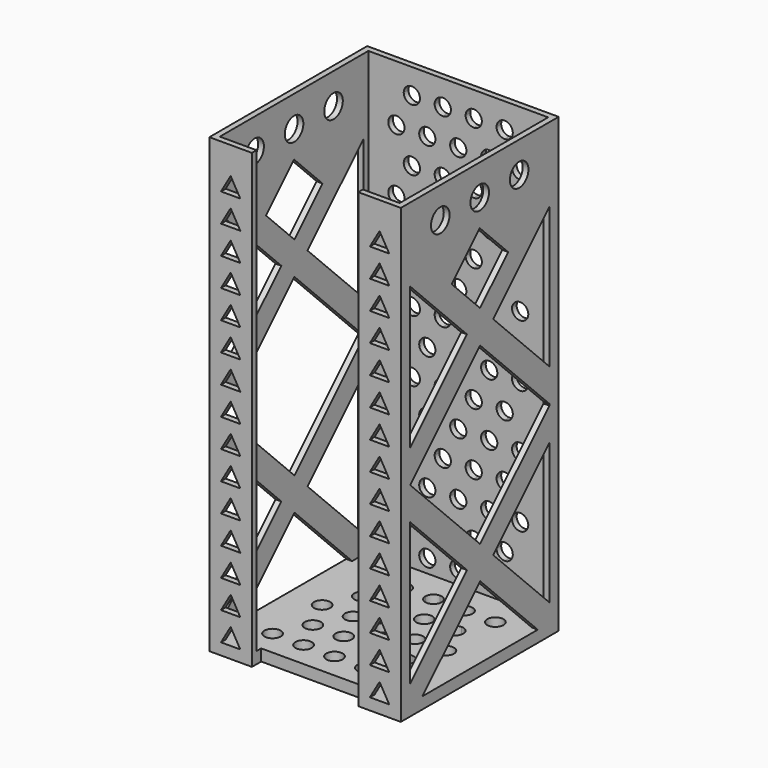
from build123d import *

# Parameters (mm, degrees)
F0_W      = 49.5
F0_H      = 51
F1_DEPTH  = 3
F2_W      = 49.5
F2_H      = 51
F2_W_2    = 46.5
F2_H_2    = 48
F3_DEPTH  = 114
F4_W      = 27.5
F4_H      = 117
F5_DEPTH  = 3
F6_R      = 2.1
F7_DEPTH  = 3
F9_DEPTH  = 106.1
F11_DEPTH = 49.501
F12_R     = 2.1
F13_DEPTH = 4
F15_DEPTH = 25


# Not quite as in the source:
# - ends of sketch curves that miss each other by under 0.0002 mm in the source are joined


with BuildPart() as f1:
    # F0 (on Top) → F1 (new body)
    with BuildSketch(Plane.XY):
        Rectangle(F0_W, F0_H)
    extrude(amount=F1_DEPTH)

    # F2 (on face) → F3 (join)
    with BuildSketch(Plane.XY.offset(3)):
        Rectangle(F2_W, F2_H)
        Rectangle(F2_W_2, F2_H_2, mode=Mode.SUBTRACT)
    extrude(amount=F3_DEPTH)

    # F4 (on face) → F5 (cut)
    with BuildSketch(Plane.XZ.offset(25.5)):
        with Locations((0, 58.5)):
            Rectangle(F4_W, F4_H)
    extrude(amount=-F5_DEPTH, mode=Mode.SUBTRACT)

    # F6 (on face) → F7 (cut)
    with BuildSketch(Plane(origin=(0, 25.5, 0), x_dir=(-1, 0, 0), z_dir=(0, 1, 0))):
        with Locations((-16, 6.5)):
            Circle(F6_R)
        with BuildLine():
            ThreePointArc((18.1, 6.5), (16, 8.6), (13.9, 6.5))
            ThreePointArc((13.9, 6.5), (16, 4.4), (18.1, 6.5))
        make_face()
        with BuildLine():
            ThreePointArc((-9.9, 14.5), (-13.4849242405, 15.9849242405), (-12, 12.4))
            ThreePointArc((-12, 12.4), (-10.5150757595, 13.0150757595), (-9.9, 14.5))
        make_face()
        with BuildLine():
            ThreePointArc((-1.9, 14.5), (-5.4849242405, 15.9849242405), (-4, 12.4))
            ThreePointArc((-4, 12.4), (-2.5150757595, 13.0150757595), (-1.9, 14.5))
        make_face()
        with BuildLine():
            ThreePointArc((6.1, 14.5), (2.5150757595, 15.9849242405), (4, 12.4))
            ThreePointArc((4, 12.4), (5.4849242405, 13.0150757595), (6.1, 14.5))
        make_face()
        with BuildLine():
            ThreePointArc((14.1, 14.5), (10.5150757595, 15.9849242405), (12, 12.4))
            ThreePointArc((12, 12.4), (13.4849242405, 13.0150757595), (14.1, 14.5))
        make_face()
        with BuildLine():
            ThreePointArc((12, 28.4), (13.4849242405, 29.0150757595), (14.1, 30.5))
            ThreePointArc((14.1, 30.5), (10.5150757595, 31.9849242405), (12, 28.4))
        make_face()
        with BuildLine():
            ThreePointArc((-1.9, 30.5), (-5.4849242405, 31.9849242405), (-4, 28.4))
            ThreePointArc((-4, 28.4), (-2.5150757595, 29.0150757595), (-1.9, 30.5))
        make_face()
        with BuildLine():
            ThreePointArc((-9.9, 30.5), (-13.4849242405, 31.9849242405), (-12, 28.4))
            ThreePointArc((-12, 28.4), (-10.5150757595, 29.0150757595), (-9.9, 30.5))
        make_face()
        with Locations((-16, 22.5)):
            Circle(F6_R)
        with BuildLine():
            ThreePointArc((6.1, 30.5), (2.5150757595, 31.9849242405), (4, 28.4))
            ThreePointArc((4, 28.4), (5.4849242405, 29.0150757595), (6.1, 30.5))
        make_face()
        with BuildLine():
            ThreePointArc((18.1, 22.5), (16, 24.6), (13.9, 22.5))
            ThreePointArc((13.9, 22.5), (16, 20.4), (18.1, 22.5))
        make_face()
        with BuildLine():
            ThreePointArc((12, 44.4), (13.4849242405, 45.0150757595), (14.1, 46.5))
            ThreePointArc((14.1, 46.5), (10.5150757595, 47.9849242405), (12, 44.4))
        make_face()
        with BuildLine():
            ThreePointArc((-1.9, 46.5), (-5.4849242405, 47.9849242405), (-4, 44.4))
            ThreePointArc((-4, 44.4), (-2.5150757595, 45.0150757595), (-1.9, 46.5))
        make_face()
        with BuildLine():
            ThreePointArc((-9.9, 46.5), (-13.4849242405, 47.9849242405), (-12, 44.4))
            ThreePointArc((-12, 44.4), (-10.5150757595, 45.0150757595), (-9.9, 46.5))
        make_face()
        with Locations((-16, 38.5)):
            Circle(F6_R)
        with BuildLine():
            ThreePointArc((6.1, 46.5), (2.5150757595, 47.9849242405), (4, 44.4))
            ThreePointArc((4, 44.4), (5.4849242405, 45.0150757595), (6.1, 46.5))
        make_face()
        with BuildLine():
            ThreePointArc((18.1, 38.5), (16, 40.6), (13.9, 38.5))
            ThreePointArc((13.9, 38.5), (16, 36.4), (18.1, 38.5))
        make_face()
        with BuildLine():
            ThreePointArc((12, 60.4), (13.4849242405, 61.0150757595), (14.1, 62.5))
            ThreePointArc((14.1, 62.5), (10.5150757595, 63.9849242405), (12, 60.4))
        make_face()
        with BuildLine():
            ThreePointArc((-1.9, 62.5), (-5.4849242405, 63.9849242405), (-4, 60.4))
            ThreePointArc((-4, 60.4), (-2.5150757595, 61.0150757595), (-1.9, 62.5))
        make_face()
        with BuildLine():
            ThreePointArc((-9.9, 62.5), (-13.4849242405, 63.9849242405), (-12, 60.4))
            ThreePointArc((-12, 60.4), (-10.5150757595, 61.0150757595), (-9.9, 62.5))
        make_face()
        with Locations((-16, 54.5)):
            Circle(F6_R)
        with BuildLine():
            ThreePointArc((6.1, 62.5), (2.5150757595, 63.9849242405), (4, 60.4))
            ThreePointArc((4, 60.4), (5.4849242405, 61.0150757595), (6.1, 62.5))
        make_face()
        with BuildLine():
            ThreePointArc((18.1, 54.5), (16, 56.6), (13.9, 54.5))
            ThreePointArc((13.9, 54.5), (16, 52.4), (18.1, 54.5))
        make_face()
        with BuildLine():
            ThreePointArc((12, 76.4), (13.4849242405, 77.0150757595), (14.1, 78.5))
            ThreePointArc((14.1, 78.5), (10.5150757595, 79.9849242405), (12, 76.4))
        make_face()
        with BuildLine():
            ThreePointArc((-1.9, 78.5), (-5.4849242405, 79.9849242405), (-4, 76.4))
            ThreePointArc((-4, 76.4), (-2.5150757595, 77.0150757595), (-1.9, 78.5))
        make_face()
        with BuildLine():
            ThreePointArc((-9.9, 78.5), (-13.4849242405, 79.9849242405), (-12, 76.4))
            ThreePointArc((-12, 76.4), (-10.5150757595, 77.0150757595), (-9.9, 78.5))
        make_face()
        with Locations((-16, 70.5)):
            Circle(F6_R)
        with BuildLine():
            ThreePointArc((6.1, 78.5), (2.5150757595, 79.9849242405), (4, 76.4))
            ThreePointArc((4, 76.4), (5.4849242405, 77.0150757595), (6.1, 78.5))
        make_face()
        with BuildLine():
            ThreePointArc((18.1, 70.5), (16, 72.6), (13.9, 70.5))
            ThreePointArc((13.9, 70.5), (16, 68.4), (18.1, 70.5))
        make_face()
        with BuildLine():
            ThreePointArc((12, 92.4), (13.4849242405, 93.0150757595), (14.1, 94.5))
            ThreePointArc((14.1, 94.5), (10.5150757595, 95.9849242405), (12, 92.4))
        make_face()
        with BuildLine():
            ThreePointArc((-1.9, 94.5), (-5.4849242405, 95.9849242405), (-4, 92.4))
            ThreePointArc((-4, 92.4), (-2.5150757595, 93.0150757595), (-1.9, 94.5))
        make_face()
        with BuildLine():
            ThreePointArc((-9.9, 94.5), (-13.4849242405, 95.9849242405), (-12, 92.4))
            ThreePointArc((-12, 92.4), (-10.5150757595, 93.0150757595), (-9.9, 94.5))
        make_face()
        with Locations((-16, 86.5)):
            Circle(F6_R)
        with BuildLine():
            ThreePointArc((6.1, 94.5), (2.5150757595, 95.9849242405), (4, 92.4))
            ThreePointArc((4, 92.4), (5.4849242405, 93.0150757595), (6.1, 94.5))
        make_face()
        with BuildLine():
            ThreePointArc((18.1, 86.5), (16, 88.6), (13.9, 86.5))
            ThreePointArc((13.9, 86.5), (16, 84.4), (18.1, 86.5))
        make_face()
        with BuildLine():
            ThreePointArc((14.1, 110.5), (10.5150757595, 111.9849242405), (12, 108.4))
            ThreePointArc((12, 108.4), (13.4849242405, 109.0150757595), (14.1, 110.5))
        make_face()
        with BuildLine():
            ThreePointArc((-9.9, 110.5), (-13.4849242405, 111.9849242405), (-12, 108.4))
            ThreePointArc((-12, 108.4), (-10.5150757595, 109.0150757595), (-9.9, 110.5))
        make_face()
        with Locations((-16, 102.5)):
            Circle(F6_R)
        with BuildLine():
            ThreePointArc((18.1, 102.5), (16, 104.6), (13.9, 102.5))
            ThreePointArc((13.9, 102.5), (16, 100.4), (18.1, 102.5))
        make_face()
        with BuildLine():
            Line((-8, 6.5), (-5.9, 6.5))
            ThreePointArc((-5.9, 6.5), (-8, 8.6), (-10.1, 6.5))
            Line((-10.1, 6.5), (-8, 6.5))
        make_face()
        with BuildLine():
            ThreePointArc((-10.1, 6.5), (-8, 4.4), (-5.9, 6.5))
            Line((-5.9, 6.5), (-8, 6.5))
            Line((-8, 6.5), (-10.1, 6.5))
        make_face()
        with BuildLine():
            ThreePointArc((10.1, 6.5), (8, 8.6), (5.9, 6.5))
            Line((5.9, 6.5), (8, 6.5))
            Line((8, 6.5), (10.1, 6.5))
        make_face()
        with BuildLine():
            Line((8, 6.5), (5.9, 6.5))
            ThreePointArc((5.9, 6.5), (8, 4.4), (10.1, 6.5))
            Line((10.1, 6.5), (8, 6.5))
        make_face()
        with BuildLine():
            Line((-8, 22.5), (-5.9, 22.5))
            ThreePointArc((-5.9, 22.5), (-8, 24.6), (-10.1, 22.5))
            Line((-10.1, 22.5), (-8, 22.5))
        make_face()
        with BuildLine():
            ThreePointArc((-10.1, 22.5), (-8, 20.4), (-5.9, 22.5))
            Line((-5.9, 22.5), (-8, 22.5))
            Line((-8, 22.5), (-10.1, 22.5))
        make_face()
        with BuildLine():
            Line((8, 22.5), (10.1, 22.5))
            ThreePointArc((10.1, 22.5), (8, 24.6), (5.9, 22.5))
            Line((5.9, 22.5), (8, 22.5))
        make_face()
        with BuildLine():
            ThreePointArc((5.9, 22.5), (8, 20.4), (10.1, 22.5))
            Line((10.1, 22.5), (8, 22.5))
            Line((8, 22.5), (5.9, 22.5))
        make_face()
        with BuildLine():
            Line((-8, 38.5), (-5.9, 38.5))
            ThreePointArc((-5.9, 38.5), (-8, 40.6), (-10.1, 38.5))
            Line((-10.1, 38.5), (-8, 38.5))
        make_face()
        with BuildLine():
            ThreePointArc((-10.1, 38.5), (-8, 36.4), (-5.9, 38.5))
            Line((-5.9, 38.5), (-8, 38.5))
            Line((-8, 38.5), (-10.1, 38.5))
        make_face()
        with BuildLine():
            Line((8, 38.5), (10.1, 38.5))
            ThreePointArc((10.1, 38.5), (8, 40.6), (5.9, 38.5))
            Line((5.9, 38.5), (8, 38.5))
        make_face()
        with BuildLine():
            ThreePointArc((5.9, 38.5), (8, 36.4), (10.1, 38.5))
            Line((10.1, 38.5), (8, 38.5))
            Line((8, 38.5), (5.9, 38.5))
        make_face()
        with BuildLine():
            Line((-8, 54.5), (-5.9, 54.5))
            ThreePointArc((-5.9, 54.5), (-8, 56.6), (-10.1, 54.5))
            Line((-10.1, 54.5), (-8, 54.5))
        make_face()
        with BuildLine():
            ThreePointArc((-10.1, 54.5), (-8, 52.4), (-5.9, 54.5))
            Line((-5.9, 54.5), (-8, 54.5))
            Line((-8, 54.5), (-10.1, 54.5))
        make_face()
        with BuildLine():
            Line((8, 54.5), (10.1, 54.5))
            ThreePointArc((10.1, 54.5), (8, 56.6), (5.9, 54.5))
            Line((5.9, 54.5), (8, 54.5))
        make_face()
        with BuildLine():
            ThreePointArc((5.9, 54.5), (8, 52.4), (10.1, 54.5))
            Line((10.1, 54.5), (8, 54.5))
            Line((8, 54.5), (5.9, 54.5))
        make_face()
        with BuildLine():
            Line((-8, 70.5), (-5.9, 70.5))
            ThreePointArc((-5.9, 70.5), (-8, 72.6), (-10.1, 70.5))
            Line((-10.1, 70.5), (-8, 70.5))
        make_face()
        with BuildLine():
            ThreePointArc((-10.1, 70.5), (-8, 68.4), (-5.9, 70.5))
            Line((-5.9, 70.5), (-8, 70.5))
            Line((-8, 70.5), (-10.1, 70.5))
        make_face()
        with BuildLine():
            Line((8, 70.5), (10.1, 70.5))
            ThreePointArc((10.1, 70.5), (8, 72.6), (5.9, 70.5))
            Line((5.9, 70.5), (8, 70.5))
        make_face()
        with BuildLine():
            ThreePointArc((5.9, 70.5), (8, 68.4), (10.1, 70.5))
            Line((10.1, 70.5), (8, 70.5))
            Line((8, 70.5), (5.9, 70.5))
        make_face()
        with BuildLine():
            Line((-8, 86.5), (-5.9, 86.5))
            ThreePointArc((-5.9, 86.5), (-8, 88.6), (-10.1, 86.5))
            Line((-10.1, 86.5), (-8, 86.5))
        make_face()
        with BuildLine():
            ThreePointArc((-10.1, 86.5), (-8, 84.4), (-5.9, 86.5))
            Line((-5.9, 86.5), (-8, 86.5))
            Line((-8, 86.5), (-10.1, 86.5))
        make_face()
        with BuildLine():
            Line((8, 86.5), (10.1, 86.5))
            ThreePointArc((10.1, 86.5), (8, 88.6), (5.9, 86.5))
            Line((5.9, 86.5), (8, 86.5))
        make_face()
        with BuildLine():
            ThreePointArc((5.9, 86.5), (8, 84.4), (10.1, 86.5))
            Line((10.1, 86.5), (8, 86.5))
            Line((8, 86.5), (5.9, 86.5))
        make_face()
        with BuildLine():
            Line((-4, 110.5), (-1.9, 110.5))
            ThreePointArc((-1.9, 110.5), (-5.4849242405, 111.9849242405), (-4, 108.4))
            Line((-4, 108.4), (-4, 110.5))
        make_face()
        with BuildLine():
            ThreePointArc((-4, 108.4), (-2.5150757595, 109.0150757595), (-1.9, 110.5))
            Line((-1.9, 110.5), (-4, 110.5))
            Line((-4, 110.5), (-4, 108.4))
        make_face()
        with BuildLine():
            Line((-8, 102.5), (-5.9, 102.5))
            ThreePointArc((-5.9, 102.5), (-8, 104.6), (-10.1, 102.5))
            Line((-10.1, 102.5), (-8, 102.5))
        make_face()
        with BuildLine():
            ThreePointArc((-10.1, 102.5), (-8, 100.4), (-5.9, 102.5))
            Line((-5.9, 102.5), (-8, 102.5))
            Line((-8, 102.5), (-10.1, 102.5))
        make_face()
        with BuildLine():
            ThreePointArc((10.1, 102.5), (8, 104.6), (5.9, 102.5))
            Line((5.9, 102.5), (8, 102.5))
            Line((8, 102.5), (10.1, 102.5))
        make_face()
        with BuildLine():
            Line((8, 102.5), (5.9, 102.5))
            ThreePointArc((5.9, 102.5), (8, 100.4), (10.1, 102.5))
            Line((10.1, 102.5), (8, 102.5))
        make_face()
        with BuildLine():
            Line((4, 110.5), (1.9, 110.5))
            ThreePointArc((1.9, 110.5), (2.5150757595, 109.0150757595), (4, 108.4))
            Line((4, 108.4), (4, 110.5))
        make_face()
        with BuildLine():
            ThreePointArc((6.1, 110.5), (4, 112.6), (1.9, 110.5))
            Line((1.9, 110.5), (4, 110.5))
            Line((4, 110.5), (4, 108.4))
            ThreePointArc((4, 108.4), (5.4849242405, 109.0150757595), (6.1, 110.5))
        make_face()
        with BuildLine():
            ThreePointArc((2.1, 6.5), (0, 8.6), (-2.1, 6.5))
            Line((-2.1, 6.5), (0, 6.5))
            Line((0, 6.5), (2.1, 6.5))
        make_face()
        with BuildLine():
            Line((0, 6.5), (-2.1, 6.5))
            ThreePointArc((-2.1, 6.5), (-1.4849242405, 5.0150757595), (0, 4.4))
            Line((0, 4.4), (0, 6.5))
        make_face()
        with BuildLine():
            Line((2.1, 6.5), (0, 6.5))
            Line((0, 6.5), (0, 4.4))
            ThreePointArc((0, 4.4), (1.4849242405, 5.0150757595), (2.1, 6.5))
        make_face()
        with BuildLine():
            ThreePointArc((0, 20.4), (1.4849242405, 21.0150757595), (2.1, 22.5))
            Line((2.1, 22.5), (0, 22.5))
            Line((0, 22.5), (0, 20.4))
        make_face()
        with BuildLine():
            Line((0, 20.4), (0, 22.5))
            Line((0, 22.5), (-2.1, 22.5))
            ThreePointArc((-2.1, 22.5), (-1.4849242405, 21.0150757595), (0, 20.4))
        make_face()
        with BuildLine():
            Line((0, 22.5), (2.1, 22.5))
            ThreePointArc((2.1, 22.5), (0, 24.6), (-2.1, 22.5))
            Line((-2.1, 22.5), (0, 22.5))
        make_face()
        with BuildLine():
            ThreePointArc((0, 36.4), (1.4849242405, 37.0150757595), (2.1, 38.5))
            Line((2.1, 38.5), (0, 38.5))
            Line((0, 38.5), (0, 36.4))
        make_face()
        with BuildLine():
            Line((0, 36.4), (0, 38.5))
            Line((0, 38.5), (-2.1, 38.5))
            ThreePointArc((-2.1, 38.5), (-1.4849242405, 37.0150757595), (0, 36.4))
        make_face()
        with BuildLine():
            Line((0, 38.5), (2.1, 38.5))
            ThreePointArc((2.1, 38.5), (0, 40.6), (-2.1, 38.5))
            Line((-2.1, 38.5), (0, 38.5))
        make_face()
        with BuildLine():
            ThreePointArc((0, 52.4), (1.4849242405, 53.0150757595), (2.1, 54.5))
            Line((2.1, 54.5), (0, 54.5))
            Line((0, 54.5), (0, 52.4))
        make_face()
        with BuildLine():
            Line((0, 52.4), (0, 54.5))
            Line((0, 54.5), (-2.1, 54.5))
            ThreePointArc((-2.1, 54.5), (-1.4849242405, 53.0150757595), (0, 52.4))
        make_face()
        with BuildLine():
            Line((0, 54.5), (2.1, 54.5))
            ThreePointArc((2.1, 54.5), (0, 56.6), (-2.1, 54.5))
            Line((-2.1, 54.5), (0, 54.5))
        make_face()
        with BuildLine():
            ThreePointArc((0, 68.4), (1.4849242405, 69.0150757595), (2.1, 70.5))
            Line((2.1, 70.5), (0, 70.5))
            Line((0, 70.5), (0, 68.4))
        make_face()
        with BuildLine():
            Line((0, 68.4), (0, 70.5))
            Line((0, 70.5), (-2.1, 70.5))
            ThreePointArc((-2.1, 70.5), (-1.4849242405, 69.0150757595), (0, 68.4))
        make_face()
        with BuildLine():
            Line((0, 70.5), (2.1, 70.5))
            ThreePointArc((2.1, 70.5), (0, 72.6), (-2.1, 70.5))
            Line((-2.1, 70.5), (0, 70.5))
        make_face()
        with BuildLine():
            ThreePointArc((0, 84.4), (1.4849242405, 85.0150757595), (2.1, 86.5))
            Line((2.1, 86.5), (0, 86.5))
            Line((0, 86.5), (0, 84.4))
        make_face()
        with BuildLine():
            Line((0, 84.4), (0, 86.5))
            Line((0, 86.5), (-2.1, 86.5))
            ThreePointArc((-2.1, 86.5), (-1.4849242405, 85.0150757595), (0, 84.4))
        make_face()
        with BuildLine():
            Line((0, 86.5), (2.1, 86.5))
            ThreePointArc((2.1, 86.5), (0, 88.6), (-2.1, 86.5))
            Line((-2.1, 86.5), (0, 86.5))
        make_face()
        with BuildLine():
            ThreePointArc((2.1, 102.5), (0, 104.6), (-2.1, 102.5))
            Line((-2.1, 102.5), (0, 102.5))
            Line((0, 102.5), (2.1, 102.5))
        make_face()
        with BuildLine():
            Line((0, 102.5), (-2.1, 102.5))
            ThreePointArc((-2.1, 102.5), (-1.4849242405, 101.0150757595), (0, 100.4))
            Line((0, 100.4), (0, 102.5))
        make_face()
        with BuildLine():
            ThreePointArc((0, 100.4), (1.4849242405, 101.0150757595), (2.1, 102.5))
            Line((2.1, 102.5), (0, 102.5))
            Line((0, 102.5), (0, 100.4))
        make_face()
    extrude(amount=-F7_DEPTH, mode=Mode.SUBTRACT)

    # F8 (on face) → F9 (cut)
    with BuildSketch(Plane.YZ.offset(24.75)):
        with BuildLine():
            Line((-3, 109), (0, 109))
            Line((0, 109), (3, 109))
            ThreePointArc((3, 109), (0, 112), (-3, 109))
        make_face()
        with BuildLine():
            Line((3, 109), (0, 109))
            Line((0, 109), (-3, 109))
            ThreePointArc((-3, 109), (0, 106), (3, 109))
        make_face()
        with BuildLine():
            ThreePointArc((15.75, 109), (12.75, 112), (9.75, 109))
            Line((9.75, 109), (15.75, 109))
        make_face()
        with BuildLine():
            Line((15.75, 109), (9.75, 109))
            ThreePointArc((9.75, 109), (12.75, 106), (15.75, 109))
        make_face()
        with BuildLine():
            ThreePointArc((-15.75, 109), (-12.75, 106), (-9.75, 109))
            Line((-9.75, 109), (-15.75, 109))
        make_face()
        with BuildLine():
            Line((-15.75, 109), (-9.75, 109))
            ThreePointArc((-9.75, 109), (-12.75, 112), (-15.75, 109))
        make_face()
    extrude(amount=-F9_DEPTH, mode=Mode.SUBTRACT)

    # F10 (on face) → F11 (cut, through all)
    with BuildSketch(Plane.YZ.offset(24.75)):
        Polygon((-4.135696358, 79.5376057473), (-22.4900200356, 97.8919294249), (-22.4900200356, 61.1832820698), align=None)
        Polygon((4.3495850162, 79.5376057473), (22.5, 61.3871907636), (22.5, 97.6880207311), align=None)
        Polygon((-22.4900200356, 52.6780407667), (0.1069443291, 30.081076402), (22.5, 52.4741320729), (22.5, 52.9019093893), (0.1069443291, 75.2949650602), (-22.4900200356, 52.6980006955), align=None)
        Polygon((-22.4900200356, 44.2453622909), (-22.4900200356, 7.4841120373), (-4.1093949088, 25.8647371641), align=None)
        Polygon((-18.5022328489, 3), (0, 3), (18.7553422553, 3), (0.1265547032, 21.6287875521), align=None)
        Polygon((4.3428939411, 25.84512679), (22.5, 7.6880207311), (22.5, 44.0022328489), align=None)
        Polygon((0, 102.0225568908), (-9.0676830636, 92.9548738272), (0, 83.8871907636), align=None)
        Polygon((0.1069443291, 83.7802464345), (9.1796173749, 92.8529194803), (0.0049899822, 102.027546873), (0, 102.0225568908), (0, 83.8871907636), align=None)
    extrude(amount=-F11_DEPTH, mode=Mode.SUBTRACT)

    # F12 (on face) → F13 (cut)
    with BuildSketch(Plane(origin=(0, 0, 0), x_dir=(1, 0, 0), z_dir=(0, 0, -1))):
        with BuildLine():
            ThreePointArc((18.1, -16), (16, -13.9), (13.9, -16))
            ThreePointArc((13.9, -16), (16, -18.1), (18.1, -16))
        make_face()
        with BuildLine():
            ThreePointArc((10.1, -16), (8, -13.9), (5.9, -16))
            Line((5.9, -16), (8, -16))
            Line((8, -16), (10.1, -16))
        make_face()
        with BuildLine():
            Line((8, -16), (5.9, -16))
            ThreePointArc((5.9, -16), (8, -18.1), (10.1, -16))
            Line((10.1, -16), (8, -16))
        make_face()
        with BuildLine():
            Line((-2.1, -16), (0, -16))
            Line((0, -16), (2.1, -16))
            ThreePointArc((2.1, -16), (0, -13.9), (-2.1, -16))
        make_face()
        with BuildLine():
            Line((0, -16), (0, -18.1))
            ThreePointArc((0, -18.1), (1.4849242405, -17.4849242405), (2.1, -16))
            Line((2.1, -16), (0, -16))
        make_face()
        with BuildLine():
            ThreePointArc((-2.1, -16), (-1.4849242405, -17.4849242405), (0, -18.1))
            Line((0, -18.1), (0, -16))
            Line((0, -16), (-2.1, -16))
        make_face()
        with BuildLine():
            ThreePointArc((-10.1, -16), (-8, -18.1), (-5.9, -16))
            Line((-5.9, -16), (-8, -16))
            Line((-8, -16), (-10.1, -16))
        make_face()
        with BuildLine():
            Line((-8, -16), (-5.9, -16))
            ThreePointArc((-5.9, -16), (-8, -13.9), (-10.1, -16))
            Line((-10.1, -16), (-8, -16))
        make_face()
        with Locations((-16, -16)):
            Circle(F12_R)
        with Locations((-12, -8)):
            Circle(F12_R)
        with BuildLine():
            ThreePointArc((-6.1, -8), (-4, -10.1), (-1.9, -8))
            Line((-1.9, -8), (-4, -8))
            Line((-4, -8), (-6.1, -8))
        make_face()
        with BuildLine():
            Line((-4, -8), (-1.9, -8))
            ThreePointArc((-1.9, -8), (-4, -5.9), (-6.1, -8))
            Line((-6.1, -8), (-4, -8))
        make_face()
        with BuildLine():
            Line((4, -8), (6.1, -8))
            ThreePointArc((6.1, -8), (4, -5.9), (1.9, -8))
            Line((1.9, -8), (4, -8))
        make_face()
        with BuildLine():
            ThreePointArc((1.9, -8), (4, -10.1), (6.1, -8))
            Line((6.1, -8), (4, -8))
            Line((4, -8), (1.9, -8))
        make_face()
        with BuildLine():
            Line((12, -8), (12, -10.1))
            ThreePointArc((12, -10.1), (13.4849242405, -9.4849242405), (14.1, -8))
            ThreePointArc((14.1, -8), (12, -5.9), (9.9, -8))
            Line((9.9, -8), (12, -8))
        make_face()
        with BuildLine():
            ThreePointArc((9.9, -8), (10.5150757595, -9.4849242405), (12, -10.1))
            Line((12, -10.1), (12, -8))
            Line((12, -8), (9.9, -8))
        make_face()
        with BuildLine():
            ThreePointArc((18.1, 0), (16, 2.1), (13.9, 0))
            ThreePointArc((13.9, 0), (16, -2.1), (18.1, 0))
        make_face()
        with BuildLine():
            Line((8, 0), (10.1, 0))
            ThreePointArc((10.1, 0), (8, 2.1), (5.9, 0))
            Line((5.9, 0), (8, 0))
        make_face()
        with BuildLine():
            ThreePointArc((5.9, 0), (8, -2.1), (10.1, 0))
            Line((10.1, 0), (8, 0))
            Line((8, 0), (5.9, 0))
        make_face()
        with BuildLine():
            ThreePointArc((-2.1, 0), (0, -2.1), (2.1, 0))
            Line((2.1, 0), (0, 0))
            Line((0, 0), (-2.1, 0))
        make_face()
        with BuildLine():
            Line((0, 0), (2.1, 0))
            ThreePointArc((2.1, 0), (0, 2.1), (-2.1, 0))
            Line((-2.1, 0), (0, 0))
        make_face()
        with BuildLine():
            Line((-8, 0), (-5.9, 0))
            ThreePointArc((-5.9, 0), (-8, 2.1), (-10.1, 0))
            Line((-10.1, 0), (-8, 0))
        make_face()
        with Locations((-16, 0)):
            Circle(F12_R)
        with Locations((-12, 8)):
            Circle(F12_R)
        with BuildLine():
            ThreePointArc((-1.9, 8), (-4, 10.1), (-6.1, 8))
            Line((-6.1, 8), (-4, 8))
            Line((-4, 8), (-1.9, 8))
        make_face()
        with BuildLine():
            Line((-4, 8), (-6.1, 8))
            ThreePointArc((-6.1, 8), (-4, 5.9), (-1.9, 8))
            Line((-1.9, 8), (-4, 8))
        make_face()
        with BuildLine():
            Line((4, 8), (1.9, 8))
            ThreePointArc((1.9, 8), (4, 5.9), (6.1, 8))
            Line((6.1, 8), (4, 8))
        make_face()
        with BuildLine():
            ThreePointArc((6.1, 8), (4, 10.1), (1.9, 8))
            Line((1.9, 8), (4, 8))
            Line((4, 8), (6.1, 8))
        make_face()
        with BuildLine():
            ThreePointArc((14.1, 8), (12, 10.1), (9.9, 8))
            Line((9.9, 8), (12, 8))
            Line((12, 8), (12, 5.9))
            ThreePointArc((12, 5.9), (13.4849242405, 6.5150757595), (14.1, 8))
        make_face()
        with BuildLine():
            Line((-16, 16), (-16, 18.1))
            ThreePointArc((-16, 18.1), (-17.4849242405, 14.5150757595), (-13.9, 16))
            Line((-13.9, 16), (-16, 16))
        make_face()
        with BuildLine():
            ThreePointArc((-13.9, 16), (-14.5150757595, 17.4849242405), (-16, 18.1))
            Line((-16, 18.1), (-16, 16))
            Line((-16, 16), (-13.9, 16))
        make_face()
        with BuildLine():
            ThreePointArc((-5.9, 16), (-8, 18.1), (-10.1, 16))
            Line((-10.1, 16), (-8, 16))
            Line((-8, 16), (-5.9, 16))
        make_face()
        with BuildLine():
            Line((-8, 16), (-10.1, 16))
            ThreePointArc((-10.1, 16), (-8, 13.9), (-5.9, 16))
            Line((-5.9, 16), (-8, 16))
        make_face()
        with BuildLine():
            ThreePointArc((2.1, 16), (0, 18.1), (-2.1, 16))
            Line((-2.1, 16), (0, 16))
            Line((0, 16), (2.1, 16))
        make_face()
        with BuildLine():
            Line((0, 16), (-2.1, 16))
            ThreePointArc((-2.1, 16), (0, 13.9), (2.1, 16))
            Line((2.1, 16), (0, 16))
        make_face()
        with BuildLine():
            ThreePointArc((10.1, 16), (8, 18.1), (5.9, 16))
            Line((5.9, 16), (8, 16))
            Line((8, 16), (10.1, 16))
        make_face()
        with BuildLine():
            Line((8, 16), (5.9, 16))
            ThreePointArc((5.9, 16), (8, 13.9), (10.1, 16))
            Line((10.1, 16), (8, 16))
        make_face()
        with BuildLine():
            ThreePointArc((18.1, 16), (16, 18.1), (13.9, 16))
            ThreePointArc((13.9, 16), (16, 13.9), (18.1, 16))
        make_face()
        with BuildLine():
            Line((12, 8), (9.9, 8))
            ThreePointArc((9.9, 8), (10.5150757595, 6.5150757595), (12, 5.9))
            Line((12, 5.9), (12, 8))
        make_face()
        with BuildLine():
            ThreePointArc((-10.1, 0), (-8, -2.1), (-5.9, 0))
            Line((-5.9, 0), (-8, 0))
            Line((-8, 0), (-10.1, 0))
        make_face()
    extrude(amount=-F13_DEPTH, mode=Mode.SUBTRACT)

    # F14 (on face) → F15 (cut)
    with BuildSketch(Plane.XZ.offset(25.5)):
        Polygon((-19.25, 109.9501270189), (-21.75, 105.62), (-19.25, 105.62), (-16.75, 105.62), align=None)
        Polygon((-19.2500550008, 102.6200317547), (-21.75, 98.29), (-19.25, 98.29), (-16.75, 98.29), align=None)
        Polygon((-19.2500550008, 95.2900317547), (-21.75, 90.96), (-19.25, 90.96), (-16.75, 90.96), align=None)
        Polygon((-19.2500550008, 87.9600317547), (-21.75, 83.63), (-19.25, 83.63), (-16.75, 83.63), align=None)
        Polygon((-19.2500550008, 80.6300317547), (-21.75, 76.3), (-19.25, 76.3), (-16.75, 76.3), align=None)
        Polygon((-19.2500550008, 73.3000317547), (-21.75, 68.97), (-19.25, 68.97), (-16.75, 68.97), align=None)
        Polygon((-19.2500550008, 65.9700317547), (-21.75, 61.64), (-19.25, 61.64), (-16.75, 61.64), align=None)
        Polygon((-19.2500550008, 58.6400317547), (-21.75, 54.31), (-19.25, 54.31), (-16.75, 54.31), align=None)
        Polygon((-19.2500550008, 51.3100317547), (-21.75, 46.98), (-19.25, 46.98), (-16.75, 46.98), align=None)
        Polygon((-19.2500550008, 43.9800317547), (-21.75, 39.65), (-19.25, 39.65), (-16.75, 39.65), align=None)
        Polygon((-19.2500550008, 36.6500317547), (-21.75, 32.32), (-19.25, 32.32), (-16.75, 32.32), align=None)
        Polygon((-19.2500550008, 29.3200317547), (-21.75, 24.99), (-19.25, 24.99), (-16.75, 24.99), align=None)
        Polygon((-19.2500550008, 21.9900317547), (-21.75, 17.66), (-19.25, 17.66), (-16.75, 17.66), align=None)
        Polygon((-21.75, 10.33), (-19.25, 10.33), (-16.75, 10.33), (-19.2499449992, 14.6600317547), align=None)
        Polygon((-19.2500550008, 7.3300317547), (-21.75, 3), (-19.25, 3), (-16.75, 3), align=None)
        Polygon((21.75, 3), (19.2500550008, 7.3300317547), (16.75, 3), (19.25, 3), align=None)
        Polygon((16.75, 10.33), (19.25, 10.33), (21.75, 10.33), (19.2500550008, 14.6600317547), align=None)
        Polygon((16.75, 17.66), (19.25, 17.66), (21.75, 17.66), (19.2500550008, 21.9900317547), align=None)
        Polygon((16.75, 24.99), (19.25, 24.99), (21.75, 24.99), (19.2500550008, 29.3200317547), align=None)
        Polygon((16.75, 32.32), (19.25, 32.32), (21.75, 32.32), (19.2500550008, 36.6500317547), align=None)
        Polygon((16.75, 39.65), (19.25, 39.65), (21.75, 39.65), (19.2500550008, 43.9800317547), align=None)
        Polygon((16.75, 46.98), (19.25, 46.98), (21.75, 46.98), (19.2500550008, 51.3100317547), align=None)
        Polygon((16.75, 54.31), (19.25, 54.31), (21.75, 54.31), (19.2500550008, 58.6400317547), align=None)
        Polygon((16.75, 61.64), (19.25, 61.64), (21.75, 61.64), (19.2500550008, 65.9700317547), align=None)
        Polygon((16.75, 68.97), (19.25, 68.97), (21.75, 68.97), (19.2500550008, 73.3000317547), align=None)
        Polygon((16.75, 76.3), (19.25, 76.3), (21.75, 76.3), (19.2500550008, 80.6300317547), align=None)
        Polygon((16.75, 83.63), (19.25, 83.63), (21.75, 83.63), (19.2500550008, 87.9600317547), align=None)
        Polygon((16.75, 90.96), (19.25, 90.96), (21.75, 90.96), (19.2500550008, 95.2900317547), align=None)
        Polygon((16.75, 98.29), (19.25, 98.29), (21.75, 98.29), (19.2500550008, 102.6200317547), align=None)
        Polygon((16.75, 105.62), (19.25, 105.62), (21.75, 105.62), (19.25, 109.9501270189), align=None)
    extrude(amount=-F15_DEPTH, mode=Mode.SUBTRACT)


solid = f1.part
